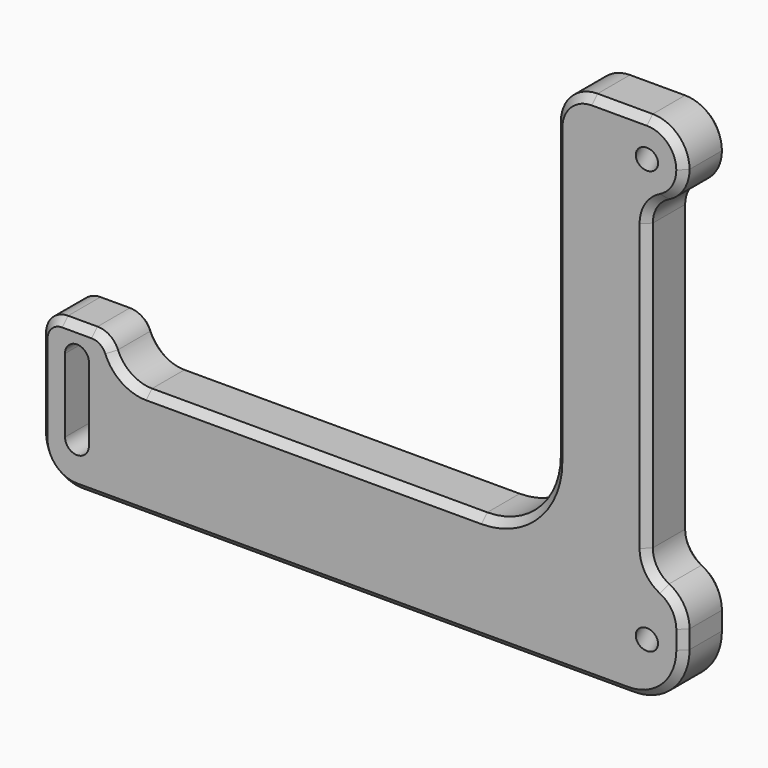
from build123d import *

# Parameters (mm, degrees)
F1_DEPTH = 15
F3_DEPTH = 20
F8_D     = 5.5
F9_R     = 8
F10_R    = 6
F11_R    = 10
F12_SIZE = 2


# Not quite as in the source:
# - ends of sketch curves that miss each other by under 0.0002 mm in the source are joined


with BuildPart() as f1:
    # F0 (on Front) → F1 (new body)
    with BuildSketch(Plane.XZ):
        with BuildLine():
            Line((-2.8333987482, 0), (-2.8333987482, 90))
            ThreePointArc((-2.8333987482, 90), (4.2344373086, 92.9306997935), (7.1616023332, 100))
            ThreePointArc((7.1616023332, 100), (4.2326701451, 107.0710678119), (-2.8383976668, 110))
            Line((-2.8383976668, 110), (-17.8333987482, 110))
            ThreePointArc((-17.8333987482, 110), (-24.9044665601, 107.0710678119), (-27.8333987482, 100))
            Line((-27.8333987482, 100), (-27.8333987482, 20))
            ThreePointArc((-27.8333987482, 20), (-33.6912631245, 5.8578643763), (-47.8333987482, 0))
            Line((-47.8333987482, 0), (-147.8333987482, 0))
            Line((-147.8333987482, 0), (-147.8333987482, 10))
            Line((-147.8333987482, 10), (-153.8333987482, 10))
            Line((-153.8333987482, 10), (-161.8333987482, 10))
            ThreePointArc((-161.8333987482, 10), (-166.0760394353, 8.2426406871), (-167.8333987482, 4))
            Line((-167.8333987482, 4), (-167.8333987482, -20))
            ThreePointArc((-167.8333987482, -20), (-164.9044665601, -27.0710678119), (-157.8333987482, -30))
            Line((-157.8333987482, -30), (-7.8333987482, -30))
            ThreePointArc((-7.8333987482, -30), (2.7732029696, -25.6066017178), (7.1666012518, -15))
            Line((7.1666012518, -15), (7.1666012518, -10))
            ThreePointArc((7.1666012518, -10), (4.2376690637, -2.9289321881), (-2.8333987482, 0))
        make_face()
    extrude(amount=F1_DEPTH)

    # F2 (on face) → F3 (cut)
    with BuildSketch(Plane.XZ.offset(15)):
        with BuildLine():
            Line((-154.5833987482, -18), (-154.5833987482, 2))
            ThreePointArc((-154.5833987482, 2), (-157.8333987482, 5.25), (-161.0833987482, 2))
            Line((-161.0833987482, 2), (-161.0833987482, -18))
            ThreePointArc((-161.0833987482, -18), (-157.8333987482, -21.25), (-154.5833987482, -18))
        make_face()
    extrude(amount=-F3_DEPTH, mode=Mode.SUBTRACT)

    # F8 (through all)
    with Locations(Plane(origin=(-9.7913406688, 20.9975978253, 0), x_dir=(-0.906307787, -0.4226182617, 0), z_dir=(-0.4226182617, 0.906307787, 0))):
        with Locations((8.9072052754, 100), (8.9072052754, -15)):
            Hole(F8_D / 2)

    # F9
    f9_edges = [f1.edges().sort_by_distance(p)[0] for p in [
        (-2.833399, -7.5, 0),
        (-2.833399, -7.5, 90),
    ]]
    fillet(f9_edges, radius=F9_R)

    # F10
    f10_edges = [f1.edges().sort_by_distance(p)[0] for p in [
        (-147.833399, -7.5, 10),
    ]]
    fillet(f10_edges, radius=F10_R)

    # F11
    f11_edges = [f1.edges().sort_by_distance(p)[0] for p in [
        (-147.833399, -7.5, 0),
    ]]
    fillet(f11_edges, radius=F11_R)

    # F12
    f12_edges = [f1.edges().sort_by_distance(p)[0] for p in [
        (-93.4172, -15, 0),
        (-93.4172, 0, 0),
        (-150.479297, 0, 8.974937),
        (-144.591172, 0, 1.708438),
        (-157.833399, 0, 10),
        (-166.076039, 0, 8.242641),
        (-33.691263, 0, 5.857864),
        (-167.833399, 0, -8),
        (-27.833399, 0, 60),
        (-164.904467, 0, -27.071068),
        (-24.904467, 0, 107.071068),
        (-82.833399, 0, -30),
        (-10.335898, 0, 110),
        (2.773203, 0, -25.606602),
        (4.23267, 0, 107.071068),
        (7.166601, 0, -12.5),
        (5.660785, 0, 94.730854),
        (5.664967, 0, -4.729537),
        (-1.632745, 0, 88.093281),
        (-1.632091, 0, 1.908145),
        (-2.833399, 0, 45.00124),
        (-150.479297, -15, 8.974937),
        (-144.591172, -15, 1.708438),
        (-157.833399, -15, 10),
        (-166.076039, -15, 8.242641),
        (-33.691263, -15, 5.857864),
        (-167.833399, -15, -8),
        (-27.833399, -15, 60),
        (-164.904467, -15, -27.071068),
        (-24.904467, -15, 107.071068),
        (-82.833399, -15, -30),
        (-10.335898, -15, 110),
        (2.773203, -15, -25.606602),
        (4.23267, -15, 107.071068),
        (7.166601, -15, -12.5),
        (5.660785, -15, 94.730854),
        (5.664967, -15, -4.729537),
        (-1.632745, -15, 88.093281),
        (-1.632091, -15, 1.908145),
        (-2.833399, -15, 45.00124),
    ]]
    chamfer(f12_edges, length=F12_SIZE)


solid = f1.part
